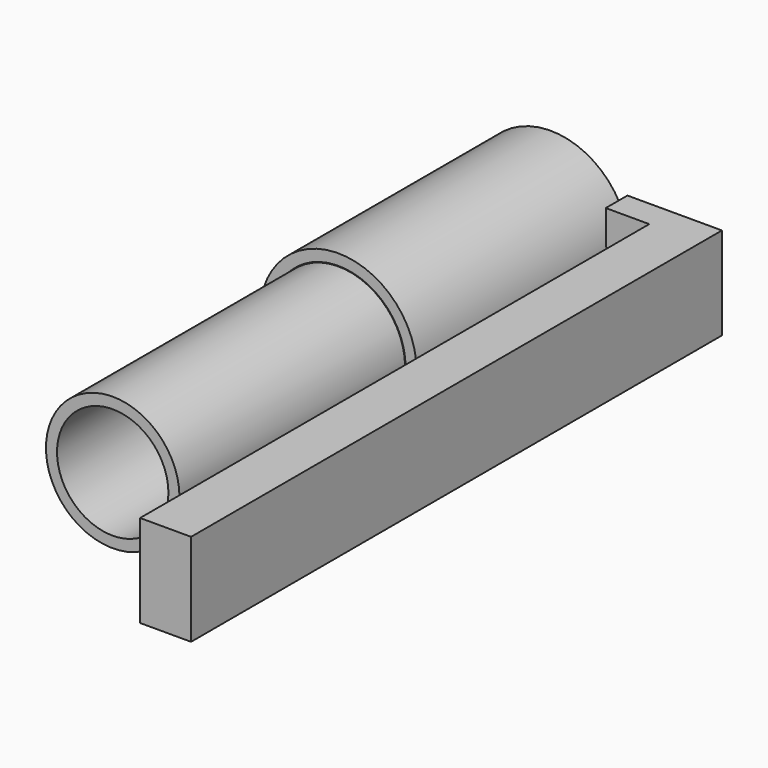
from build123d import *

# Parameters (mm, degrees)
F0_R      = 5.3975
F1_DEPTH  = 18.288
F2_T      = -0.762
F3_R      = 4.600211285
F4_DEPTH  = 19.431
F5_T      = -0.762
F6_W      = 4.6940159253
F6_H      = 10.2641077222
F7_DEPTH  = 45.72
F8_W      = 3.4673514045
F8_H      = 45.72
F9_DEPTH  = 25.4
F10_W     = 45.72
F10_H     = 1.9464063645
F10_H_2   = 1.9479215399
F11_DEPTH = 25.4
F12_W     = 1.8670405261
F12_H     = 6.3697798178
F13_DEPTH = 5.2832
F14_W     = 43.8529594739
F14_H     = 6.3697798178
F15_DEPTH = 2.286


with BuildPart() as f1:
    # F0 (on Front) → F1 (new body)
    with BuildSketch(Plane.XZ):
        Circle(F0_R)
    extrude(amount=F1_DEPTH)

    # F2
    f2_openings = [f1.faces().sort_by_distance(p)[0] for p in [
        (0, 0, 0),
        (0, -18.288, 0),
    ]]
    offset(amount=F2_T, openings=f2_openings)


with BuildPart() as f4:
    # F3 (on face) → F4 (new body)
    with BuildSketch(Plane.XZ.offset(18.288)):
        Circle(F3_R)
    extrude(amount=F4_DEPTH)

    # F5
    f5_openings = [f4.faces().sort_by_distance(p)[0] for p in [
        (0, -37.719, 0),
        (0, -18.288, 0),
    ]]
    offset(amount=F5_T, openings=f5_openings)


with BuildPart() as f7:
    # F6 (on face) → F7 (new body)
    with BuildSketch(Plane(origin=(0, 0, 0), x_dir=(-1, 0, 0), z_dir=(0, 1, 0))):
        with Locations((-9.4523209978, -0.0007575877)):
            Rectangle(F6_W, F6_H)
    extrude(amount=-F7_DEPTH)

    # F8 (on face) → F9 (cut)
    with BuildSketch(Plane(origin=(0, 0, -5.1328114488), x_dir=(1, 0, 0), z_dir=(0, 0, -1))):
        with Locations((8.8389887374, 22.86)):
            Rectangle(F8_W, F8_H)
    extrude(amount=-F9_DEPTH, mode=Mode.SUBTRACT)

    # F10 (on face) → F11 (cut)
    with BuildSketch(Plane.YZ.offset(11.7993289605)):
        with Locations((-22.86, 4.1580930911)):
            Rectangle(F10_W, F10_H)
        with Locations((-22.86, -4.1588506788)):
            Rectangle(F10_W, F10_H_2)
    extrude(amount=-F11_DEPTH, mode=Mode.SUBTRACT)

    # F12 (on face) → F13 (join)
    with BuildSketch(Plane(origin=(10.5726644397, 0, 0), x_dir=(0, -1, 0), z_dir=(-1, 0, 0))):
        with Locations((0.9335202631, 0)):
            Rectangle(F12_W, F12_H)
    extrude(amount=F13_DEPTH)

    # F14 (on face) → F15 (join)
    with BuildSketch(Plane(origin=(10.5726644397, 0, 0), x_dir=(0, -1, 0), z_dir=(-1, 0, 0))):
        with Locations((23.7935202631, 0)):
            Rectangle(F14_W, F14_H)
    extrude(amount=F15_DEPTH)


solid = Compound([f1.part, f4.part, f7.part])
